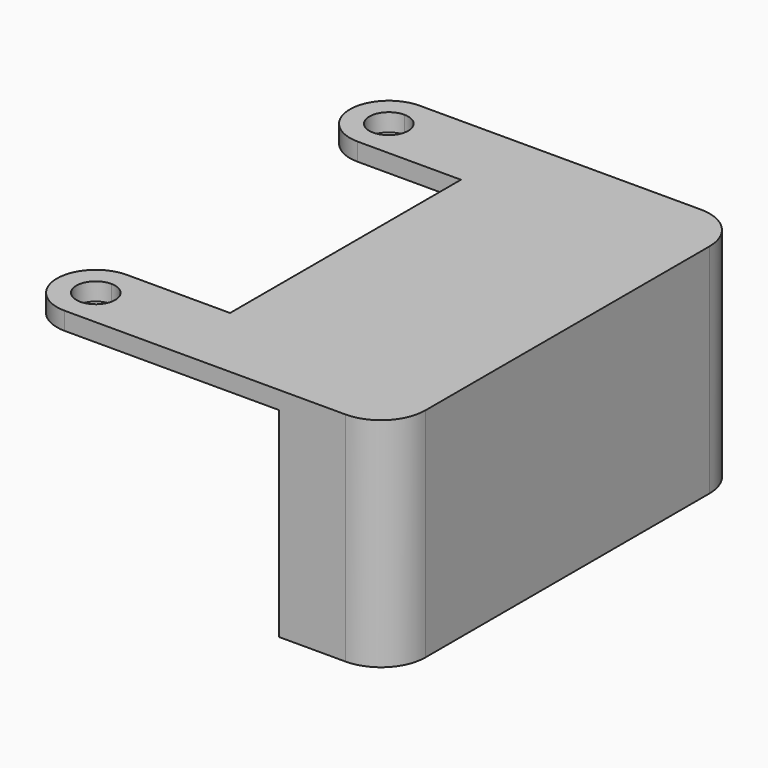
from build123d import *

# Parameters (mm, degrees)
F1_DEPTH = 1.6
F2_DEPTH = 18
F3_R     = 4
F4_R     = 2


# Not quite as in the source:
# - a feature names something its author has since deleted; it is built from what else it names


with BuildPart() as f1:
    # F0 (on Top) → F1 (new body)
    with BuildSketch(Plane.XY):
        with BuildLine():
            Line((-9.3, 18.25), (-9.3, 20))
            ThreePointArc((-9.3, 20), (-12.8, 16.5), (-9.3, 13))
            Line((-9.3, 13), (-9.3, 14.75))
            ThreePointArc((-9.3, 14.75), (-11.05, 16.5), (-9.3, 18.25))
        make_face()
        with BuildLine():
            ThreePointArc((-5.8, 16.5), (-6.8251262658, 18.9748737342), (-9.3, 20))
            Line((-9.3, 20), (-9.3, 18.25))
            ThreePointArc((-9.3, 18.25), (-8.0625631329, 17.7374368671), (-7.55, 16.5))
            ThreePointArc((-7.55, 16.5), (-8.0625631329, 15.2625631329), (-9.3, 14.75))
            Line((-9.3, 14.75), (-9.3, 13))
            ThreePointArc((-9.3, 13), (-6.8251262658, 14.0251262658), (-5.8, 16.5))
        make_face()
        with BuildLine():
            Line((0, 13), (0, 20))
            Line((0, 20), (-9.3, 20))
            ThreePointArc((-9.3, 20), (-6.8251262658, 18.9748737342), (-5.8, 16.5))
            ThreePointArc((-5.8, 16.5), (-6.8251262658, 14.0251262658), (-9.3, 13))
            Line((-9.3, 13), (0, 13))
        make_face()
        with BuildLine():
            Line((-9.3, -14.75), (-9.3, -13))
            ThreePointArc((-9.3, -13), (-12.8, -16.5), (-9.3, -20))
            Line((-9.3, -20), (-9.3, -18.25))
            ThreePointArc((-9.3, -18.25), (-11.05, -16.5), (-9.3, -14.75))
        make_face()
        with BuildLine():
            ThreePointArc((-5.8, -16.5), (-6.8251262658, -14.0251262658), (-9.3, -13))
            Line((-9.3, -13), (-9.3, -14.75))
            ThreePointArc((-9.3, -14.75), (-8.0625631329, -15.2625631329), (-7.55, -16.5))
            ThreePointArc((-7.55, -16.5), (-8.0625631329, -17.7374368671), (-9.3, -18.25))
            Line((-9.3, -18.25), (-9.3, -20))
            ThreePointArc((-9.3, -20), (-6.8251262658, -18.9748737342), (-5.8, -16.5))
        make_face()
        with BuildLine():
            Line((0, -20), (0, -13))
            Line((0, -13), (-9.3, -13))
            ThreePointArc((-9.3, -13), (-6.8251262658, -14.0251262658), (-5.8, -16.5))
            ThreePointArc((-5.8, -16.5), (-6.8251262658, -18.9748737342), (-9.3, -20))
            Line((-9.3, -20), (0, -20))
        make_face()
        Polygon((2, 18), (0, 20), (0, 13), (0, -13), (0, -20), (2, -18), align=None)
        Polygon((20, 20), (10, 20), (10, 18), (18, 18), (18, -18), (10, -18), (10, -20), (20, -20), align=None)
        Polygon((10, 18), (2, 18), (2, -18), (10, -18), (18, -18), (18, 18), align=None)
        Polygon((10, 20), (0, 20), (2, 18), (10, 18), align=None)
        Polygon((10, -18), (2, -18), (0, -20), (10, -20), align=None)
    extrude(amount=F1_DEPTH)

    # F0 (on Top) → F2 (join)
    with BuildSketch(Plane.XY):
        Polygon((20, 20), (10, 20), (10, 18), (18, 18), (18, -18), (10, -18), (10, -20), (20, -20), align=None)
    extrude(amount=-F2_DEPTH)

    # F3
    f3_edges = [f1.edges().sort_by_distance(p)[0] for p in [
        (20, -20, -8.2),
        (20, 20, -8.2),
    ]]
    fillet(f3_edges, radius=F3_R)

    # F4
    f4_edges = [f1.edges().sort_by_distance(p)[0] for p in [
        (18, -18, -9),
        (18, 18, -9),
    ]]
    fillet(f4_edges, radius=F4_R)


solid = f1.part
